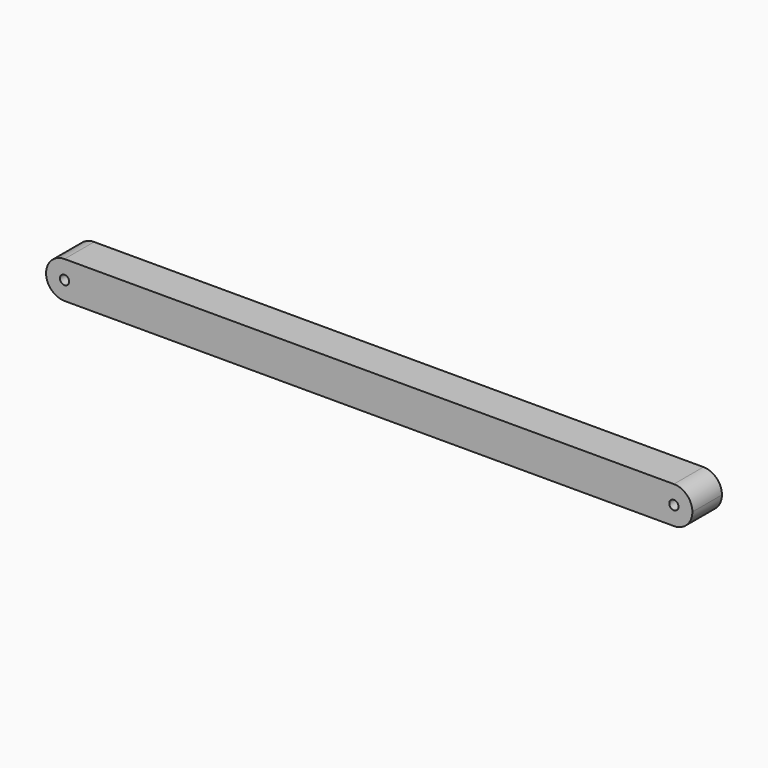
from build123d import *

# Parameters (mm, degrees)
F0_W     = 111.07674
F0_H     = 6.35
F0_R     = 0.79375
F1_DEPTH = 6.35
F2_R     = 3.17499


# Not quite as in the source:
# - a fillet or chamfer is up to 0.001 mm smaller than in the source, because OpenCascade refuses the exact size


with BuildPart() as f1:
    # F0 (on Front) → F1 (new body)
    with BuildSketch(Plane.XZ):
        with Locations((0, 3.175)):
            Rectangle(F0_W, F0_H)
        with Locations((-52.36337, 3.175)):
            Circle(F0_R, mode=Mode.SUBTRACT)
        with Locations((52.36337, 3.175)):
            Circle(F0_R, mode=Mode.SUBTRACT)
    extrude(amount=F1_DEPTH)

    # F2 (radius 3.175 in the source; OpenCascade refuses exactly that, so slightly less here)
    f2_edges = [f1.edges().sort_by_distance(p)[0] for p in [
        (55.53837, -3.175, 6.35),
        (55.53837, -3.175, 0),
        (-55.53837, -3.175, 6.35),
        (-55.53837, -3.175, 0),
    ]]
    fillet(f2_edges, radius=F2_R)


solid = f1.part
